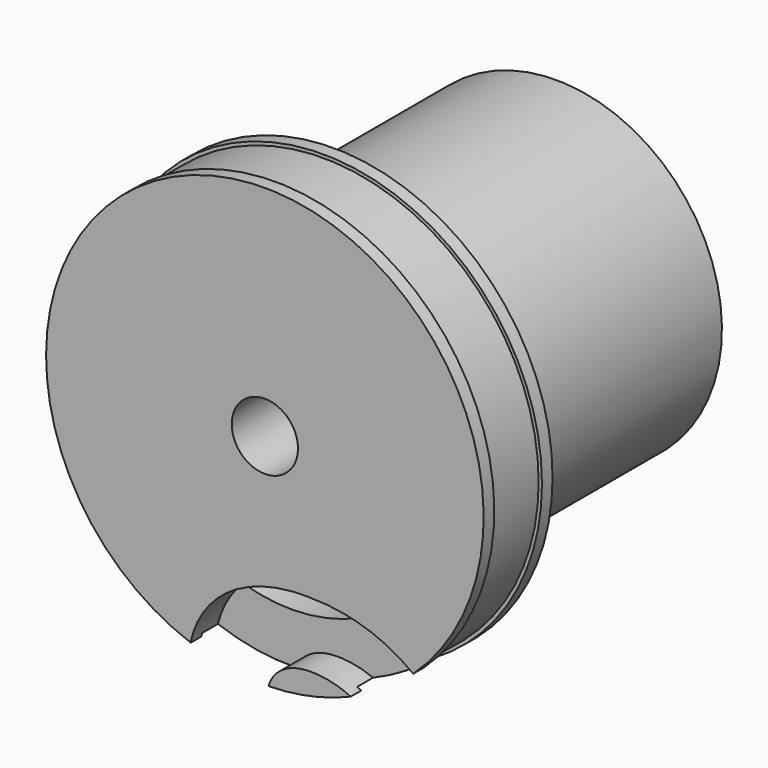
from build123d import *

# Parameters (mm, degrees)
F0_W         = 5
F0_H         = 10
F2_R         = 1.75
F3_DEPTH     = 80
F4_TEXT_SIZE = 76.1800963018
F5_DEPTH     = 25
F6_TEXT_SIZE = 78.0381443393
F7_DEPTH     = 25
F2_R_2       = 5
F9_DEPTH     = 25
F10_R        = 5
F11_DEPTH    = 50


# Not quite as in the source:
# - Text() gives the source's letters only with a copy of the font that has no kerning and outlines rounded to 1/6400 em; it was checked with that copy


with BuildPart() as f1:
    # F0 (on Top) → F1 (revolve)
    with BuildSketch(Plane.XY):
        with Locations((2.5, 10)):
            Rectangle(F0_W, F0_H)
        Polygon((0, 0), (0.6282398701, 0), (33.0282398701, 0), (33.0282398701, 2), (32.5282398701, 2), (32.5282398701, 11), (33.0282398701, 11), (33.0282398701, 13), (25.0282398701, 13), (25.0282398701, 5), (5, 5), (0, 5), align=None)
    revolve(axis=Axis((0, 10, 0), (0, 1, 0)))

    # F2 (on face) → F3 (cut)
    with BuildSketch(Plane(origin=(0, 15, 0), x_dir=(-1, 0, 0), z_dir=(0, 1, 0))):
        Circle(F2_R)
    extrude(amount=-F3_DEPTH, mode=Mode.SUBTRACT)

    # F4 (on face) → F5 (cut)
    with BuildSketch(Plane(origin=(0, 5, 0), x_dir=(-1, 0, 0), z_dir=(0, 1, 0))):
        with Locations((-121.7395216227, 36.4549681544)):
            Text('SÚPER', F4_TEXT_SIZE, font='Open Sans', font_style=FontStyle.BOLD, text_align=(TextAlign.LEFT, TextAlign.BOTTOM))
    extrude(amount=-F5_DEPTH, mode=Mode.SUBTRACT)

    # F6 (on face) → F7 (cut)
    with BuildSketch(Plane(origin=(0, 5, 0), x_dir=(-1, 0, 0), z_dir=(0, 1, 0))):
        with Locations((-28.9862323552, -75.7029093802)):
            Text("21'", F6_TEXT_SIZE, font='Open Sans', font_style=FontStyle.BOLD, text_align=(TextAlign.LEFT, TextAlign.BOTTOM))
    extrude(amount=-F7_DEPTH, mode=Mode.SUBTRACT)

    # F2 (on face) → F9 (cut)
    with BuildSketch(Plane(origin=(0, 15, 0), x_dir=(-1, 0, 0), z_dir=(0, 1, 0))):
        Circle(F2_R_2)
        Circle(F2_R, mode=Mode.SUBTRACT)
        Circle(F2_R)
    extrude(amount=-F9_DEPTH, mode=Mode.SUBTRACT)

    # F10 (on face) → F11 (join)
    with BuildSketch(Plane(origin=(0, 5, 0), x_dir=(-1, 0, 0), z_dir=(0, 1, 0))):
        with BuildLine():
            ThreePointArc((7.2441056821, -23.9274514495), (20.0761381004, -14.8979421053), (25, 0))
            ThreePointArc((25, 0), (-11.4228986944, 22.2377468602), (-14.5613908335, -20.321562366))
            add(Edge.make_bspline(
                [(7.2441056821, -23.9274514495), (5.4897102472, -22.2396564691), (-0.9046938531, -19.1984154945), (-10.0863692731, -19.1984154945), (-13.9343673843, -20.1365940816), (-14.5613908335, -20.321562366)],
                knots=[4.6051504947, 4.6051504947, 4.6051504947, 5.2911392405, 6.4367088608, 7.3065923341, 7.4824872488, 7.4824872488, 7.4824872488], degree=2))
        make_face()
        Circle(F10_R, mode=Mode.SUBTRACT)
    extrude(amount=F11_DEPTH)


solid = f1.part
